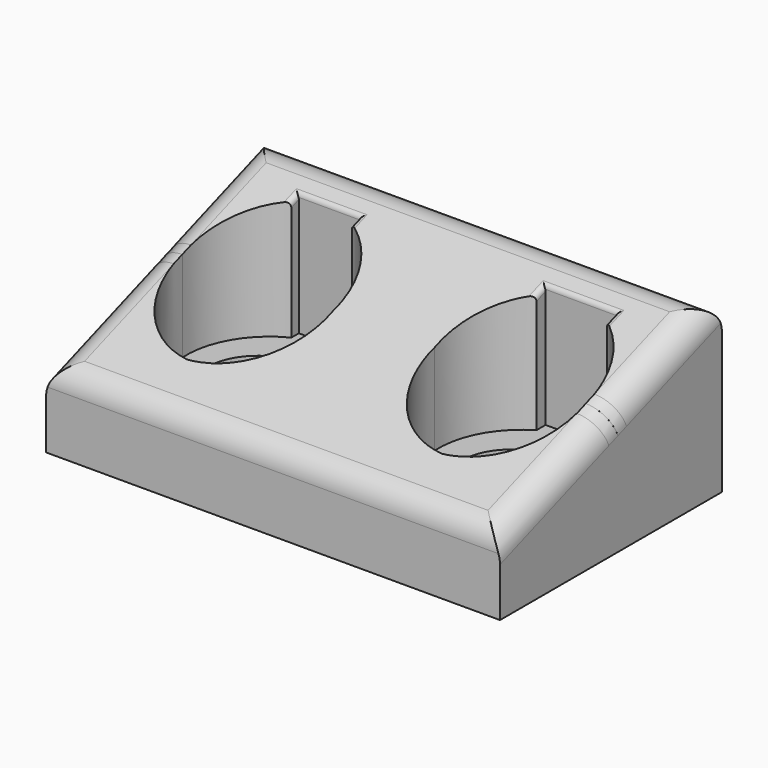
from build123d import *

# Parameters (mm, degrees)
F0_W     = 90
F0_H     = 55
F1_DEPTH = 35
F2_DEPTH = 7
F3_R     = 10
F4_DEPTH = 5
F6_DEPTH = 90
F7_R     = 4.99999
F8_W     = 12
F8_H     = 3
F9_DEPTH = 30.7
F10_R    = 1


# Not quite as in the source:
# - a fillet or chamfer is up to 0.001 mm smaller than in the source, because OpenCascade refuses the exact size
# - a feature names something its author has since deleted; it is built from what else it names


with BuildPart() as f1:
    # F0 (on Top) → F1 (new body)
    with BuildSketch(Plane.XY):
        Rectangle(F0_W, F0_H)
        with BuildLine():
            ThreePointArc((-40, 0), (-36.0621543344, 11.8032751438), (-25, 17.5))
            ThreePointArc((-25, 17.5), (-13.9378456656, 11.8032751438), (-10, 0))
            ThreePointArc((-10, 0), (-13.9378456656, -11.8032751438), (-25, -17.5))
            ThreePointArc((-25, -17.5), (-36.0621543344, -11.8032751438), (-40, 0))
        make_face(mode=Mode.SUBTRACT)
        with BuildLine():
            ThreePointArc((10, 0), (13.9500894873, 11.8143319509), (25.0340790777, 17.5))
            ThreePointArc((25.0340790777, 17.5), (36.0744106495, 11.7922476991), (40, 0))
            ThreePointArc((40, 0), (36.2593265414, -11.6306402206), (25.5441482581, -17.5))
            ThreePointArc((25.5441482581, -17.5), (14.1318309156, -11.9833988689), (10, 0))
        make_face(mode=Mode.SUBTRACT)
    extrude(amount=F1_DEPTH)

    # F0 (on Top) → F2 (join)
    with BuildSketch(Plane.XY):
        with BuildLine():
            ThreePointArc((-10, 0), (-13.9378456656, 11.8032751438), (-25, 17.5))
            ThreePointArc((-25, 17.5), (-36.0621543344, 11.8032751438), (-40, 0))
            ThreePointArc((-40, 0), (-36.0621543344, -11.8032751438), (-25, -17.5))
            ThreePointArc((-25, -17.5), (-13.9378456656, -11.8032751438), (-10, 0))
        make_face()
        with BuildLine():
            ThreePointArc((40, 0), (36.0744106495, 11.7922476991), (25.0340790777, 17.5))
            ThreePointArc((25.0340790777, 17.5), (13.9500894873, 11.8143319509), (10, 0))
            ThreePointArc((10, 0), (14.1318309156, -11.9833988689), (25.5441482581, -17.5))
            ThreePointArc((25.5441482581, -17.5), (36.2593265414, -11.6306402206), (40, 0))
        make_face()
    extrude(amount=F2_DEPTH)

    # F3 (on face) → F4 (cut)
    with BuildSketch(Plane.XY.offset(7)):
        with Locations((-25, 0)):
            Circle(F3_R)
        with Locations((25.2891136679, 0)):
            Circle(F3_R)
    extrude(amount=-F4_DEPTH, mode=Mode.SUBTRACT)

    # F5 (on face) → F6 (cut)
    with BuildSketch(Plane.YZ.offset(45)):
        Polygon((-27.5, 15), (27.5, 35), (-27.5, 35), align=None)
    extrude(amount=-F6_DEPTH, mode=Mode.SUBTRACT)

    # F7 (radius 5 in the source; OpenCascade refuses exactly that, so slightly less here)
    f7_edges = [f1.edges().sort_by_distance(p)[0] for p in [
        (0, 27.5, 35),
        (-45, 0, 25),
        (0, -27.5, 15),
        (45, 0, 25),
    ]]
    fillet(f7_edges, radius=F7_R)

    # F8 (on face) → F9 (cut)
    with BuildSketch(Plane.XY.offset(7)):
        with Locations((-24.9983986142, 16.138614808)):
            Rectangle(F8_W, F8_H)
        Polygon((32.0340790777, 17.5), (25.0340790777, 17.5), (18.0340790777, 17.5), (18.0340790777, 14.5), (32.0340790777, 14.5), align=None)
    extrude(amount=F9_DEPTH, mode=Mode.SUBTRACT)

    # F10
    f10_edges = [f1.edges().sort_by_distance(p)[0] for p in [
        (-24.998399, 17.638615, 31.414042),
        (-30.998399, 16.709549, 31.0762),
        (-18.998399, 16.708736, 31.075904),
        (32.034079, 16.355367, 30.947406),
        (25.034079, 17.5, 31.363636),
        (18.034079, 16.372599, 30.953672),
    ]]
    fillet(f10_edges, radius=F10_R)


solid = f1.part
